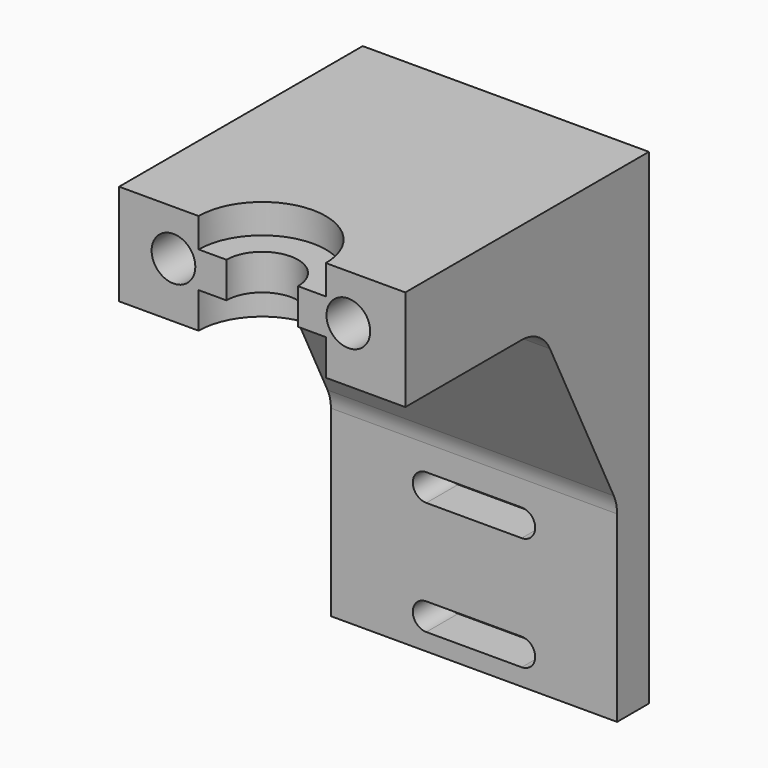
from build123d import *

# Parameters (mm, degrees)
F0_W      = 30
F0_H      = 22
F1_DEPTH  = 5
F2_DEPTH  = 39.1
F3_W      = 30
F3_H      = 12.7
F4_DEPTH  = 50
F8_W      = 30
F8_H      = 5
F9_DEPTH  = 25
F10_W     = 30
F10_H     = 5
F11_DEPTH = 5
F12_W     = 30
F12_H     = 5
F13_DEPTH = 25
F15_DEPTH = 25
F16_DEPTH = 3
F18_DEPTH = 3
F19_DEPTH = 3
F21_DEPTH = 3
F23_DEPTH = 30
F24_R     = 2.75
F25_DEPTH = 500
F26_W     = 68.0921077728
F26_H     = 72.8289508261
F27_DEPTH = 25
F29_DEPTH = 36
F30_R     = 4.99999
F32_DEPTH = 1
F33_W     = 82.302633673
F33_H     = 75.4934260622
F34_DEPTH = 50


# Not quite as in the source:
# - a fillet or chamfer is up to 0.001 mm smaller than in the source, because OpenCascade refuses the exact size


with BuildPart() as f1:
    # F0 (on Front) → F1 (new body)
    with BuildSketch(Plane.XZ):
        with Locations((0, 7.15)):
            Rectangle(F0_W, F0_H)
        with BuildLine():
            ThreePointArc((-6, -1.7), (-7.7, 0), (-6, 1.7))
            Line((-6, 1.7), (6, 1.7))
            ThreePointArc((6, 1.7), (7.7, 0), (6, -1.7))
            Line((6, -1.7), (-6, -1.7))
        make_face(mode=Mode.SUBTRACT)
        with BuildLine():
            ThreePointArc((-6, 12.6), (-7.7, 14.3), (-6, 16))
            Line((-6, 16), (6, 16))
            ThreePointArc((6, 16), (7.7, 14.3), (6, 12.6))
            Line((6, 12.6), (-6, 12.6))
        make_face(mode=Mode.SUBTRACT)
    extrude(amount=F1_DEPTH)

    # F2 (add): a face of the model
    f2_faces = [f1.faces().sort_by_distance(p)[0] for p in [
        (0, -2.5, 18.15),
    ]]
    extrude(f2_faces, amount=F2_DEPTH)

    # F3 (on face) → F4 (join)
    with BuildSketch(Plane.XZ.offset(5)):
        with Locations((0, 50.9)):
            Rectangle(F3_W, F3_H)
    extrude(amount=F4_DEPTH)

    # F6 (on offset) → F7 (revolve, cut)
    with BuildSketch(Plane.XZ.offset(38.3)):
        Polygon((8, 57.25), (0, 57.25), (0, 44.55), (8, 44.55), (8, 49.05), (4.5, 49.05), (4.5, 53.55), (8, 53.55), align=None)
    revolve(axis=Axis((0, -38.3, 50.9), (0, 0, 1)), mode=Mode.SUBTRACT)

    # F8 (on face) → F9 (join)
    with BuildSketch(Plane(origin=(0, 0, 0), x_dir=(-1, 0, 0), z_dir=(0, 1, 0))):
        with Locations((0, 36.45)):
            Rectangle(F8_W, F8_H)
    extrude(amount=F9_DEPTH)

    # F10 (on face) → F11 (join)
    with BuildSketch(Plane(origin=(0, 0, 33.95), x_dir=(1, 0, 0), z_dir=(0, 0, -1))):
        with Locations((0, -22.5)):
            Rectangle(F10_W, F10_H)
    extrude(amount=F11_DEPTH)

    # F12 (on face) → F13 (join)
    with BuildSketch(Plane(origin=(0, 25, 0), x_dir=(-1, 0, 0), z_dir=(0, 1, 0))):
        with Locations((0, 31.45)):
            Rectangle(F12_W, F12_H)
    extrude(amount=F13_DEPTH)

    # F14 (on face) → F15 (cut)
    with BuildSketch(Plane.XY.offset(33.95)):
        with BuildLine():
            ThreePointArc((7.4548611111, 38.3216117173), (0, 45), (-7.4548611111, 38.3216117173))
            ThreePointArc((-7.4548611111, 38.3216117173), (-10.75, 37.5), (-7.4548611111, 36.6783882827))
            ThreePointArc((-7.4548611111, 36.6783882827), (0, 30), (7.4548611111, 36.6783882827))
            ThreePointArc((7.4548611111, 36.6783882827), (10.75, 37.5), (7.4548611111, 38.3216117173))
        make_face()
    extrude(amount=-F15_DEPTH, mode=Mode.SUBTRACT)

    # F16 (add): a face of the model
    f16_faces = [f1.faces().sort_by_distance(p)[0] for p in [
        (15, -2.5, -2.6351662665),
    ]]
    extrude(f16_faces, amount=F16_DEPTH)

    # F17 (on face) → F18 (join)
    with BuildSketch(Plane.YZ.offset(18)):
        Polygon((50, 33.95), (0, 57.25), (0, 38.95), (25, 38.95), (25, 33.95), align=None)
    extrude(amount=-F18_DEPTH)

    # F19 (add): a face of the model
    f19_faces = [f1.faces().sort_by_distance(p)[0] for p in [
        (-15, -2.5, -2.6351662665),
    ]]
    extrude(f19_faces, amount=F19_DEPTH)

    # F20 (on face) → F21 (join)
    with BuildSketch(Plane(origin=(-18, 0, 0), x_dir=(0, -1, 0), z_dir=(-1, 0, 0))):
        Polygon((0, 57.25), (-50, 33.95), (-25, 33.95), (-25, 38.95), (0, 38.95), align=None)
    extrude(amount=-F21_DEPTH)

    # F22 (on face) → F23 (join, through all)
    with BuildSketch(Plane(origin=(15, 0, 0), x_dir=(0, -1, 0), z_dir=(-1, 0, 0))):
        Polygon((-25, 45.6), (-25, 38.95), (0, 38.95), (0, 57.25), align=None)
    extrude(amount=F23_DEPTH)

    # F24 (on face) → F25 (cut)
    with BuildSketch(Plane.XZ.offset(55)):
        with Locations((-11.1628601777, 51.5)):
            Circle(F24_R)
        with Locations((10.8371398223, 51.5)):
            Circle(F24_R)
    extrude(amount=-F25_DEPTH, mode=Mode.SUBTRACT)

    # F26 (on offset) → F27 (cut)
    with BuildSketch(Plane.XZ.offset(38.3)):
        with Locations((0.2960525453, 29.3092119973)):
            Rectangle(F26_W, F26_H)
    extrude(amount=F27_DEPTH, mode=Mode.SUBTRACT)

    # F28 (on face) → F29 (join)
    with BuildSketch(Plane(origin=(-18, 0, 0), x_dir=(0, -1, 0), z_dir=(-1, 0, 0))):
        Polygon((5, 44.55), (5, 20.35), (16.9268529862, 44.55), align=None)
    extrude(amount=-F29_DEPTH)

    # F30 (radius 5 in the source; OpenCascade refuses exactly that, so slightly less here)
    f30_edges = [f1.edges().sort_by_distance(p)[0] for p in [
        (0, -16.926853, 44.55),
        (0, 20, 33.95),
        (0, -5, 20.35),
    ]]
    fillet(f30_edges, radius=F30_R)

    # F31 (on face) → F32 (cut)
    with BuildSketch(Plane(origin=(-18, 0, 0), x_dir=(0, -1, 0), z_dir=(-1, 0, 0))):
        with BuildLine():
            ThreePointArc((2.083333126, 43.103029569), (2.7667506365, 41.4531137462), (4.4166664593, 40.7696962357))
            Line((4.4166664593, 40.7696962357), (11.4166664593, 40.7696962357))
            ThreePointArc((11.4166664593, 40.7696962357), (13.0665822821, 41.4531137462), (13.7499997926, 43.103029569))
            Line((13.7499997926, 43.103029569), (13.7499997926, 50.103029569))
            ThreePointArc((13.7499997926, 50.103029569), (13.0665822821, 51.7529453918), (11.4166664593, 52.4363629023))
            Line((11.4166664593, 52.4363629023), (4.4166664593, 52.4363629023))
            ThreePointArc((4.4166664593, 52.4363629023), (2.7667506365, 51.7529453918), (2.083333126, 50.103029569))
            Line((2.083333126, 50.103029569), (2.083333126, 43.103029569))
        make_face()
        with BuildLine():
            Line((9.6666664593, 43.103029569), (6.1666664593, 43.103029569))
            ThreePointArc((6.1666664593, 43.103029569), (4.9292295922, 43.6155927019), (4.4166664593, 44.853029569))
            Line((4.4166664593, 44.853029569), (4.4166664593, 48.353029569))
            ThreePointArc((4.4166664593, 48.353029569), (4.9292295922, 49.5904664361), (6.1666664593, 50.103029569))
            Line((6.1666664593, 50.103029569), (9.6666664593, 50.103029569))
            ThreePointArc((9.6666664593, 50.103029569), (10.9041033264, 49.5904664361), (11.4166664593, 48.353029569))
            Line((11.4166664593, 48.353029569), (11.4166664593, 44.853029569))
            ThreePointArc((11.4166664593, 44.853029569), (11.3861769533, 44.5277855668), (11.2957708468, 44.2138747406))
            Line((11.2957708593, 44.2138747357), (8.8241202093, 46.6855253857))
            ThreePointArc((8.8241201983, 46.6855253747), (8.4116412426, 46.8563797523), (7.9991622869, 46.6855253747))
            Line((7.999162276, 46.6855253857), (7.9166664593, 46.603029569))
            Line((7.9166664593, 46.603029569), (7.8341706426, 46.5205337523))
            ThreePointArc((7.8341706536, 46.5205337413), (7.663316276, 46.1080547857), (7.8341706536, 45.69557583))
            Line((7.8341706426, 45.695575819), (10.3058212926, 43.223925169))
            ThreePointArc((10.3058212877, 43.2239251815), (9.9919104615, 43.133519075), (9.6666664593, 43.103029569))
        make_face(mode=Mode.SUBTRACT)
    extrude(amount=-F32_DEPTH, mode=Mode.SUBTRACT)

    # F33 (on face) → F34 (cut)
    with BuildSketch(Plane(origin=(0, 50, 0), x_dir=(-1, 0, 0), z_dir=(0, 1, 0))):
        with Locations((4.7368425876, 23.2401336543)):
            Rectangle(F33_W, F33_H)
        Polygon((-18, 33.95), (-15, 33.95), (15, 33.95), (18, 33.95), (18, 28.95), (-18, 28.95), align=None, mode=Mode.SUBTRACT)
        Polygon((15, 33.95), (-15, 33.95), (-18, 33.95), (-18, 28.95), (18, 28.95), (18, 33.95), align=None)
    extrude(amount=-F34_DEPTH, mode=Mode.SUBTRACT)


solid = f1.part
